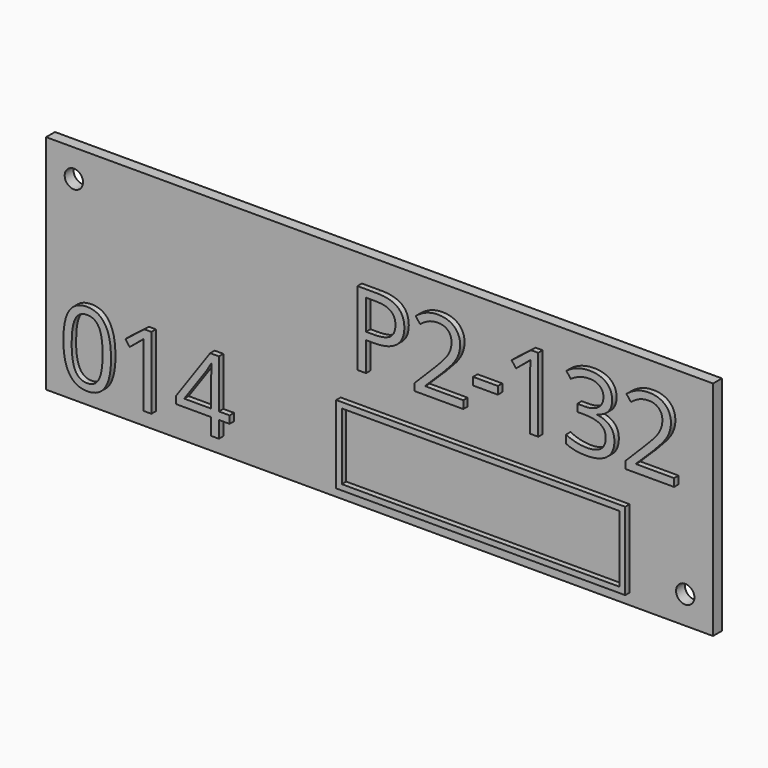
from build123d import *

# Parameters (mm, degrees)
F0_W         = 120
F0_H         = 40
F1_DEPTH     = 2
F3_D         = 3.3
F4_TEXT_SIZE = 18.6226964113
F5_DEPTH     = 1
F6_TEXT_SIZE = 18.1818181818
F7_DEPTH     = 1
F8_W         = 52
F8_H         = 14
F8_W_2       = 49.99999962
F8_H_2       = 11.99999962
F9_DEPTH     = 1


# Not quite as in the source:
# - Text() gives the source's letters only with a copy of the font that has no kerning and outlines rounded to 1/6400 em; it was checked with that copy


with BuildPart() as f1:
    # F0 (on Front) → F1 (new body)
    with BuildSketch(Plane.XZ):
        Rectangle(F0_W, F0_H)
    extrude(amount=F1_DEPTH)

    # F3 (through all)
    with Locations(Plane.XZ.offset(2)):
        with Locations((-55, 15), (55, -15)):
            Hole(F3_D / 2)

    # F4 (on face) → F5 (join)
    with BuildSketch(Plane.XZ.offset(2)):
        with Locations((-5, 2)):
            Text('P2-132', F4_TEXT_SIZE, font='Open Sans', text_align=(TextAlign.LEFT, TextAlign.BOTTOM))
    extrude(amount=F5_DEPTH)

    # F6 (on face) → F7 (join)
    with BuildSketch(Plane.XZ.offset(2)):
        with Locations((-57, -17)):
            Text('014', F6_TEXT_SIZE, font='Open Sans', text_align=(TextAlign.LEFT, TextAlign.BOTTOM))
    extrude(amount=F7_DEPTH)

    # F8 (on face) → F9 (join)
    with BuildSketch(Plane.XZ.offset(2)):
        with Locations((19, -11)):
            Rectangle(F8_W, F8_H)
        with Locations((19, -11)):
            Rectangle(F8_W_2, F8_H_2, mode=Mode.SUBTRACT)
    extrude(amount=F9_DEPTH)


solid = f1.part
